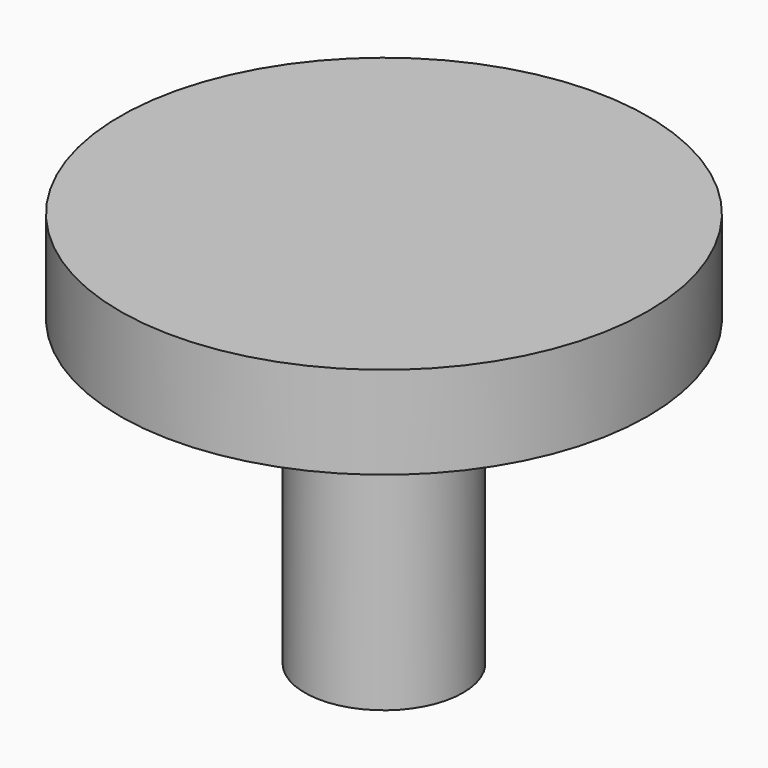
from build123d import *

# Parameters (mm, degrees)
F0_R     = 0.762
F1_DEPTH = 3.81
F2_R     = 2.54
F3_DEPTH = 0.635
F4_R     = 1.143
F4_R_2   = 0.762
F5_DEPTH = 0.5588
F6_DEPTH = 0.254


with BuildPart() as f1:
    # F0 (on Top) → F1 (new body)
    with BuildSketch(Plane.XY):
        Circle(F0_R)
    extrude(amount=F1_DEPTH)

    # F2 (on face) → F3 (join)
    with BuildSketch(Plane.XY.offset(3.81)):
        Circle(F2_R)
    extrude(amount=-F3_DEPTH)

    # F4 (on face) → F5 (cut)
    with BuildSketch(Plane(origin=(0, 0, 3.175), x_dir=(1, 0, 0), z_dir=(0, 0, -1))):
        Circle(F4_R)
        Circle(F4_R_2, mode=Mode.SUBTRACT)
    extrude(amount=-F5_DEPTH, mode=Mode.SUBTRACT)

    # F6 (add): a face of the model
    f6_faces = [f1.faces().sort_by_distance(p)[0] for p in [
        (-2.468157951, 0, 3.175),
    ]]
    extrude(f6_faces, amount=F6_DEPTH)


solid = f1.part
